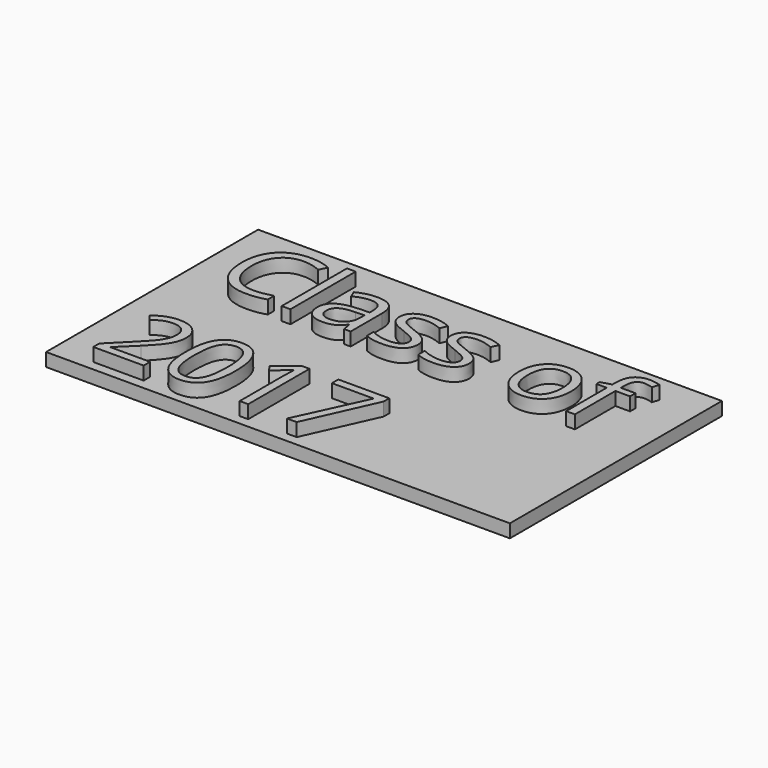
from build123d import *

# Parameters (mm, degrees)
F0_W         = 70
F0_H         = 40
F1_DEPTH     = 2
F2_TEXT_SIZE = 16.1956980177
F3_DEPTH     = 4


# Not quite as in the source:
# - Text() gives the source's letters only with a copy of the font that has no kerning and outlines rounded to 1/6400 em; it was checked with that copy


with BuildPart() as f1:
    # F0 (on Top) → F1 (new body)
    with BuildSketch(Plane.XY):
        with Locations((35, -20)):
            Rectangle(F0_W, F0_H)
    extrude(amount=F1_DEPTH)

    # F2 (on Top) → F3 (join)
    with BuildSketch(Plane.XY):
        with Locations((5.1480745498, -16.4928646)):
            Text('Class of', F2_TEXT_SIZE, font='Open Sans', text_align=(TextAlign.LEFT, TextAlign.BOTTOM))
        with Locations((5.1480745498, -38.5190139041)):
            Text('2017', F2_TEXT_SIZE, font='Open Sans', text_align=(TextAlign.LEFT, TextAlign.BOTTOM))
    extrude(amount=F3_DEPTH)


solid = f1.part
